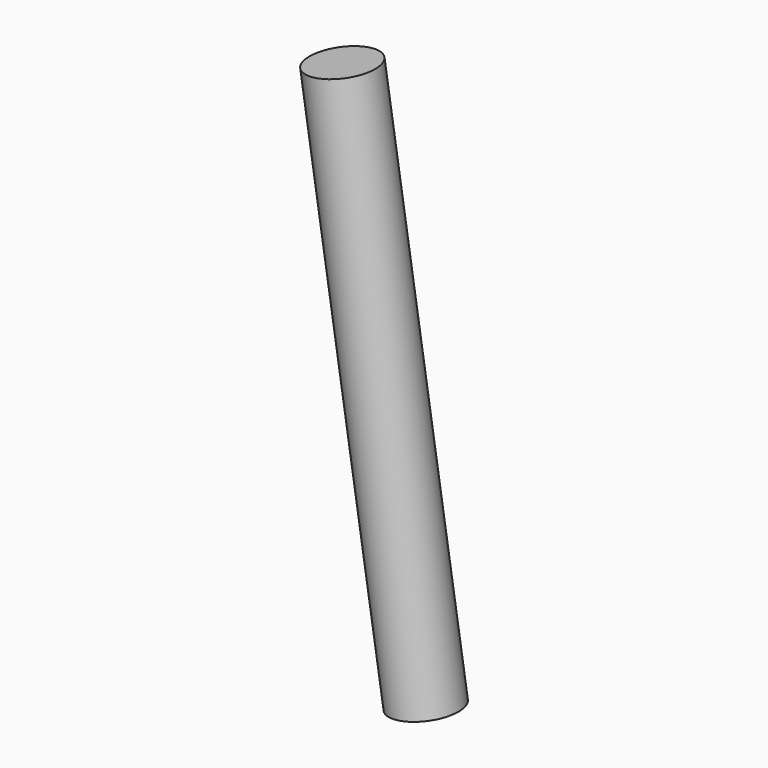
from build123d import *

# Parameters (mm, degrees)
F2_R = 50.8


with BuildPart() as f3:
    # F3: sweep along a path in F0
    with BuildLine(Plane.XZ) as f3_path:
        Line((97.700672204, 139.5514710159), (225.27, -684.22))
    # F2 (on face) → F3 (sweep)
    with BuildSketch(Plane(origin=(44.9679880436, 0, -290.3781520159), x_dir=(0.9882206238, 0, 0.1530359391), z_dir=(0.1530359391, 0, -0.9882206238))):
        with Locations((117.9062096564, 0)):
            Circle(F2_R)
    sweep(path=f3_path.line)


solid = f3.part
